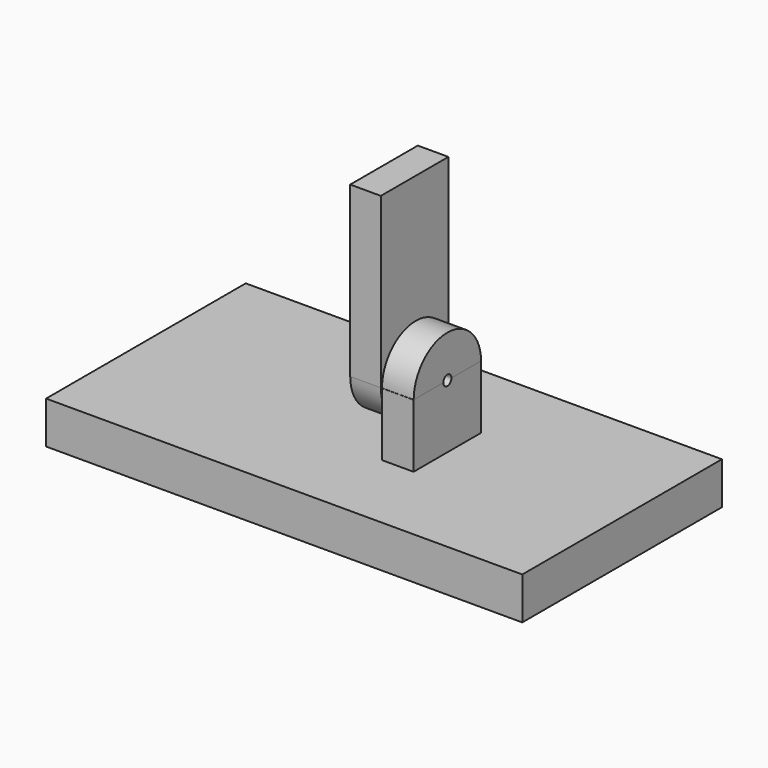
from build123d import *

# Parameters (mm, degrees)
F0_W      = 45.1033711433
F0_H      = 23.637060076
F1_DEPTH  = 4
F2_W      = 3
F2_H      = 8
F3_DEPTH  = 6
F5_DEPTH  = 3
F6_DEPTH  = 4
F7_W      = 2.9
F7_H      = 16
F8_DEPTH  = 8
F10_DEPTH = 2.9
F11_DEPTH = 9


with BuildPart() as f1:
    # F0 (on Top) → F1 (new body)
    with BuildSketch(Plane.XY):
        Rectangle(F0_W, F0_H)
    extrude(amount=F1_DEPTH)

    # F2 (on face) → F3 (join)
    with BuildSketch(Plane.XY.offset(4)):
        with Locations((4.5, 0)):
            Rectangle(F2_W, F2_H)
    extrude(amount=F3_DEPTH)

    # F4 (on face) → F6 (cut)
    with BuildSketch(Plane.YZ.offset(6)):
        with BuildLine():
            ThreePointArc((-0.4757382244, 10), (0, 9.5242617756), (0.4757382244, 10))
            Line((0.4757382244, 10), (-0.4757382244, 10))
        make_face()
    extrude(amount=-F6_DEPTH, mode=Mode.SUBTRACT)


with BuildPart() as f5:
    # F4 (on face) → F5 (new body)
    with BuildSketch(Plane.YZ.offset(6)):
        with BuildLine():
            Line((0.4757382244, 10), (3.9853850795, 10))
            ThreePointArc((3.9853850795, 10), (0, 13.9853850795), (-3.9853850795, 10))
            Line((-3.9853850795, 10), (-0.4757382244, 10))
            ThreePointArc((-0.4757382244, 10), (0, 10.4757382244), (0.4757382244, 10))
        make_face()
    extrude(amount=-F5_DEPTH)


with BuildPart() as f8:
    # F7 (on face) → F8 (new body)
    with BuildSketch(Plane.XZ.offset(4)):
        with Locations((1.45, 18)):
            Rectangle(F7_W, F7_H)
    extrude(amount=-F8_DEPTH)

    # F9 (on face) → F10 (join)
    with BuildSketch(Plane(origin=(0, 0, 0), x_dir=(0, -1, 0), z_dir=(-1, 0, 0))):
        with BuildLine():
            Line((0.7107497932, 10), (4, 10))
            ThreePointArc((4, 10), (0, 14), (-4, 10))
            Line((-4, 10), (-0.7107497932, 10))
            ThreePointArc((-0.7107497932, 10), (0, 10.7107497932), (0.7107497932, 10))
        make_face()
        with BuildLine():
            ThreePointArc((-4, 10), (0, 6), (4, 10))
            Line((4, 10), (0.7107497932, 10))
            ThreePointArc((0.7107497932, 10), (0, 9.2892502068), (-0.7107497932, 10))
            Line((-0.7107497932, 10), (-4, 10))
        make_face()
    extrude(amount=-F10_DEPTH)

    # F9 (on face) → F11 (cut)
    with BuildSketch(Plane(origin=(0, 0, 0), x_dir=(0, -1, 0), z_dir=(-1, 0, 0))):
        with BuildLine():
            ThreePointArc((-0.7107497932, 10), (0, 9.2892502068), (0.7107497932, 10))
            Line((0.7107497932, 10), (-0.7107497932, 10))
        make_face()
        with BuildLine():
            Line((-0.7107497932, 10), (0.7107497932, 10))
            ThreePointArc((0.7107497932, 10), (0, 10.7107497932), (-0.7107497932, 10))
        make_face()
    extrude(amount=-F11_DEPTH, mode=Mode.SUBTRACT)


solid = Compound([f1.part, f5.part, f8.part])
